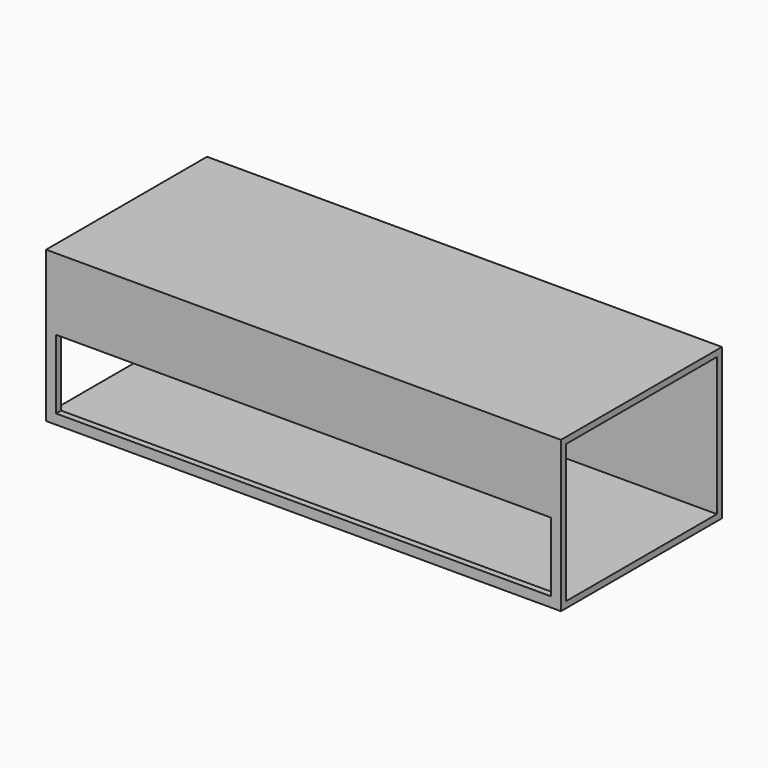
from build123d import *

# Parameters (mm, degrees)
F0_W     = 101.6
F0_H     = 76.2
F0_W_2   = 95.25
F0_H_2   = 69.85
F1_DEPTH = 130
F2_W     = 250
F2_H     = 35
F3_DEPTH = 3.175


with BuildPart() as f1:
    # F0 (on Right) → F1 (new body, symmetric)
    with BuildSketch(Plane.YZ):
        Rectangle(F0_W, F0_H)
        Rectangle(F0_W_2, F0_H_2, mode=Mode.SUBTRACT)
    extrude(amount=F1_DEPTH, both=True)

    # F2 (on face) → F3 (cut, through all)
    with BuildSketch(Plane.XZ.offset(50.8)):
        with Locations((0, -15.6)):
            Rectangle(F2_W, F2_H)
    extrude(amount=-F3_DEPTH, mode=Mode.SUBTRACT)


solid = f1.part
